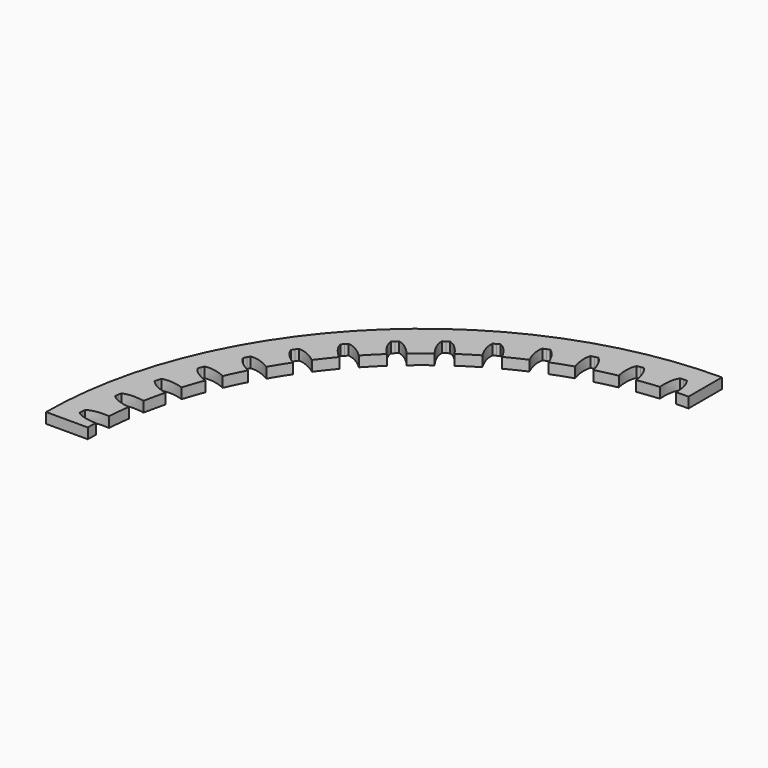
from build123d import *

# Parameters (mm, degrees)
F1_DEPTH        = 12.7
F3_DEPTH        = 12.701
F3_COPIES_COUNT = 14
F3_COPIES_ANGLE = 83.5714285714


# Not quite as in the source:
# - a pattern or mirror of a feature is missing from the dataset's text; its kind, count and spacing are read off the source's solid


with BuildPart() as f1:
    # F0 (on Top) → F1 (new body)
    with BuildSketch(Plane.XY):
        with BuildLine():
            Line((0, 406.4), (0, 457.2))
            ThreePointArc((0, 457.2), (-323.2892203585, 323.2892203585), (-457.2, 0))
            Line((-457.2, 0), (-406.4, 0))
            ThreePointArc((-406.4, 0), (-287.3681958742, 287.3681958742), (0, 406.4))
        make_face()
    extrude(amount=F1_DEPTH)

    # F2 (on face) → F3 (cut, through all)
    with BuildSketch(Plane.XY.offset(12.7)):
        with BuildLine():
            ThreePointArc((-431.208233107, 22.5986659057), (-431.307308063, 20.6214939188), (-431.3973173561, 18.643888488))
            add(Edge.make_bspline(
                [(-431.3973173561, 18.643888488), (-430.2147687313, 17.7620058271), (-426.8500319292, 15.4790427408), (-418.1275807876, 12.5466064043), (-409.1569871203, 11.7796169074), (-406.2261352346, 11.8864230253)],
                knots=[0, 0, 0, 0, 0.2583833756, 0.6107568534, 1, 1, 1, 1], degree=3))
            ThreePointArc((-406.2261352346, 11.8864230253), (-406.061691467, 16.5789843773), (-405.8430429243, 21.2693326171))
            ThreePointArc((-405.8430429243, 21.2693326171), (-405.5702187937, 25.9568416347), (-405.2432554943, 30.640885699))
            add(Edge.make_bspline(
                [(-430.9828947268, 26.5515433249), (-429.7146423877, 27.3049849498), (-426.1297033427, 29.2237309583), (-417.1485116373, 31.2283586879), (-408.1468875873, 31.0534641654), (-405.2432554943, 30.640885699)],
                knots=[0, 0, 0, 0, 0.2583833756, 0.6107568534, 1, 1, 1, 1], degree=3))
            ThreePointArc((-430.9828947268, 26.5515433249), (-431.1000945706, 24.5753628905), (-431.208233107, 22.5986659057))
        make_face()
    f3 = extrude(amount=-F3_DEPTH, mode=Mode.SUBTRACT)

    # F3_copies: F3 ×14 about axis
    f3_copies_axis = Axis((0, 0, 0), (0, 0, -1))
    for i in range(1, F3_COPIES_COUNT):
        add(f3.rotate(f3_copies_axis, i * F3_COPIES_ANGLE / (F3_COPIES_COUNT - 1)), mode=Mode.SUBTRACT)


solid = f1.part
